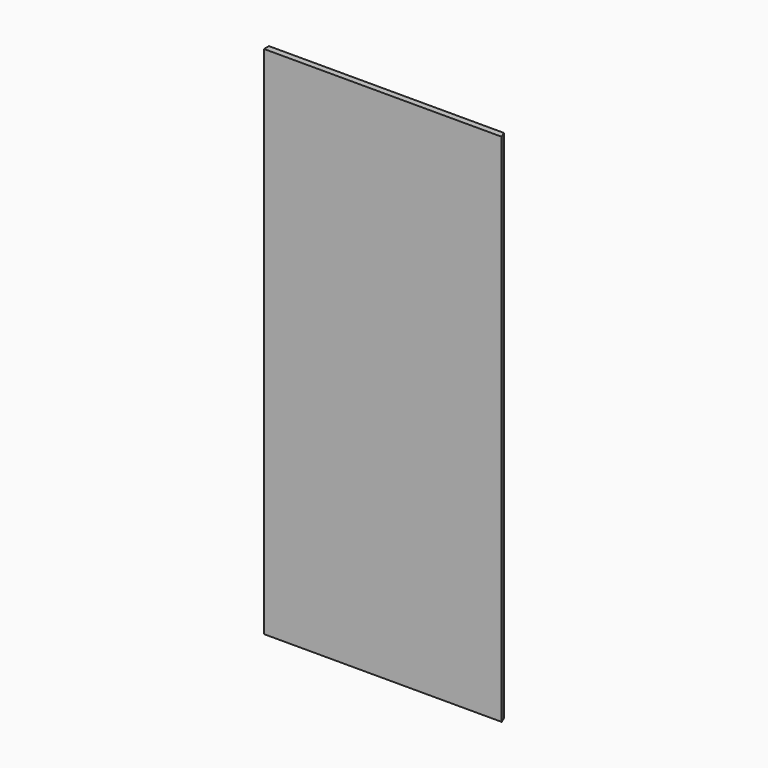
from build123d import *

# Parameters (mm, degrees)
F0_W     = 486.3619122421
F0_H     = 1054.1
F1_DEPTH = 12.7
F2_SIZE2 = 5.260502
F2_SIZE  = 12.69999


# Not quite as in the source:
# - a fillet or chamfer is up to 0.001 mm smaller than in the source, because OpenCascade refuses the exact size


with BuildPart() as f1:
    # F0 (on Front) → F1 (new body)
    with BuildSketch(Plane.XZ):
        with Locations((243.1809561211, 527.05)):
            Rectangle(F0_W, F0_H)
    extrude(amount=-F1_DEPTH)

    # F2 (size 12.7 and 5.2605122421 in the source; OpenCascade refuses exactly that, so slightly less here)
    f2_edges = [f1.edges().sort_by_distance(p)[0] for p in [
        (486.361912, 12.7, 527.05),
    ]]
    f2_side = f1.faces().sort_by_distance((486.361912, 6.35, 527.05))[0]
    chamfer(f2_edges, length=F2_SIZE, length2=F2_SIZE2, reference=f2_side)


solid = f1.part
